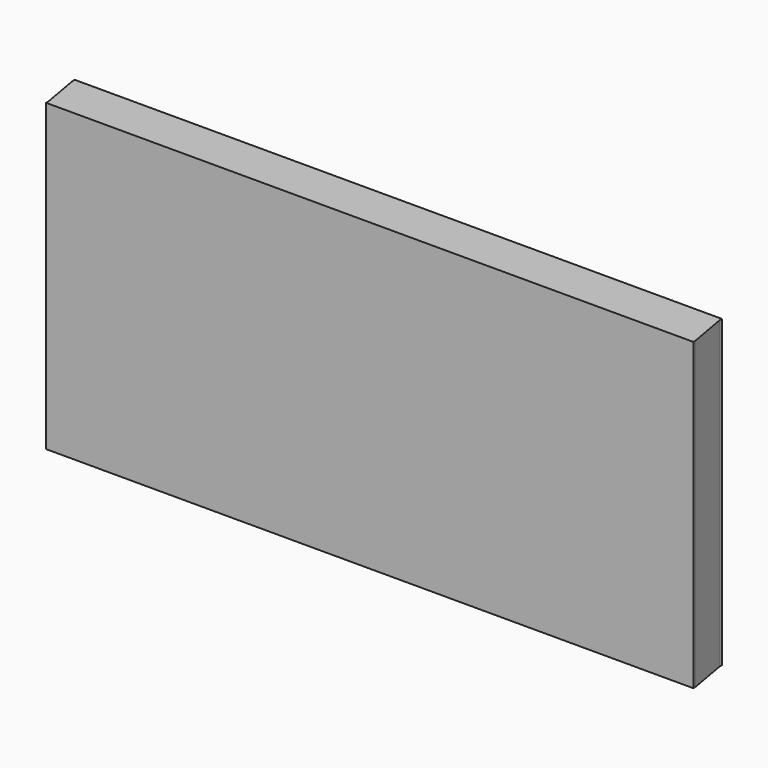
from build123d import *

# Parameters (mm, degrees)
F0_W     = 198.9582
F0_H     = 622.3
F0_W_2   = 221.1972716
F1_DEPTH = 88.9
F3_DEPTH = 698.5
F5_DEPTH = 698.501
F6_W     = 1482.6882716
F6_H     = 698.5
F7_DEPTH = 6.35
F8_W     = 1482.6882716
F8_H     = 698.5
F9_DEPTH = 6.35


# Not quite as in the source:
# - a feature names something its author has since deleted; it is built from what else it names


with BuildPart() as f1:
    # F0 (on Front) → F1 (new body)
    with BuildSketch(Plane.XZ):
        Polygon((0, 38.1), (0, 0), (1482.6882716, 0), (1482.6882716, 38.1), (1482.6882716, 660.4), (1482.6882716, 698.5), (0, 698.5), (0, 660.4), align=None)
        with Locations((137.5791, 349.25)):
            Rectangle(F0_W, F0_H, mode=Mode.SUBTRACT)
        with Locations((374.6373, 349.25)):
            Rectangle(F0_W, F0_H, mode=Mode.SUBTRACT)
        with Locations((611.6955, 349.25)):
            Rectangle(F0_W, F0_H, mode=Mode.SUBTRACT)
        with Locations((848.7537, 349.25)):
            Rectangle(F0_W, F0_H, mode=Mode.SUBTRACT)
        with Locations((1085.8119, 349.25)):
            Rectangle(F0_W, F0_H, mode=Mode.SUBTRACT)
        with Locations((1333.9896358, 349.25)):
            Rectangle(F0_W_2, F0_H, mode=Mode.SUBTRACT)
    extrude(amount=F1_DEPTH)

    # F2 (on face) → F3 (join, through all)
    with BuildSketch(Plane.XY.offset(698.5)):
        Polygon((-15.675468585, 0), (0, -88.9), (0, 0), align=None)
    extrude(amount=-F3_DEPTH)

    # F4 (on face) → F5 (cut, through all)
    with BuildSketch(Plane.XY.offset(698.5)):
        Polygon((1467.012803015, 0), (1482.6882716, -88.9), (1482.6882716, 0), align=None)
    extrude(amount=-F5_DEPTH, mode=Mode.SUBTRACT)

    # F6 (on face) → F7 (join)
    with BuildSketch(Plane.XZ.offset(88.9)):
        with Locations((741.3441358, 349.25)):
            Rectangle(F6_W, F6_H)
    extrude(amount=F7_DEPTH)

    # F8 (on face) → F9 (join)
    with BuildSketch(Plane(origin=(0, 0, 0), x_dir=(-1, 0, 0), z_dir=(0, 1, 0))):
        with Locations((-725.668667215, 349.25)):
            Rectangle(F8_W, F8_H)
    extrude(amount=F9_DEPTH)


solid = f1.part
